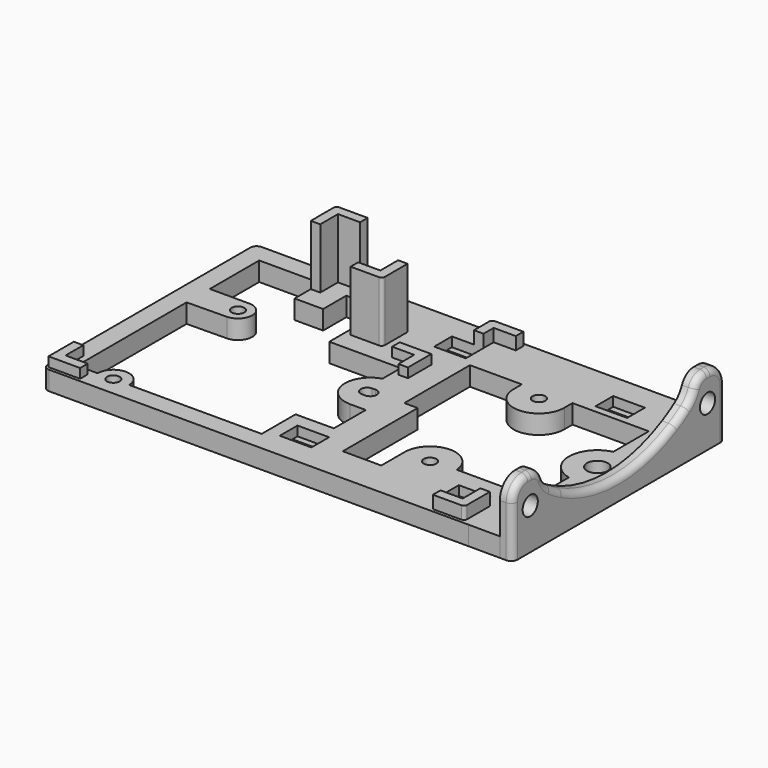
from build123d import *

# Parameters (mm, degrees)
F0_R      = 2
F0_R_2    = 3.3
F1_DEPTH  = 6
F2_DEPTH  = 10
F3_R      = 3
F4_DEPTH  = 4
F5_R      = 5
F6_R      = 5
F7_R      = 6
F8_R      = 6
F9_DEPTH  = 25
F0_W      = 10
F0_H      = 2
F10_DEPTH = 3
F11_R     = 2
F12_R     = 1
F14_DEPTH = 9


# Not quite as in the source:
# - two fillets or chamfers of one size are made in one step
# - a feature names something its author has since deleted; it is built from what else it names


with BuildPart() as f1:
    # F0 (on Top) → F1 (new body)
    with BuildSketch(Plane.XY):
        with BuildLine():
            Line((-86.7564441767, -23.0754980175), (-72.2564441767, -23.0754980175))
            Line((-72.2564441767, -23.0754980175), (47.7435558233, -23.0754980175))
            Line((47.7435558233, -23.0754980175), (57.7435558233, -23.1136400253))
            Line((57.7435558233, -23.1136400253), (57.7435558233, 60.9245019825))
            Line((57.7435558233, 60.9245019825), (47.7435558233, 60.9245019825))
            Line((47.7435558233, 60.9245019825), (-51.2561814487, 60.9245019825))
            Line((-51.2561814487, 60.9245019825), (-51.2561814487, 57.9245019825))
            Line((-51.2561814487, 57.9245019825), (-58.2561814487, 57.9245019825))
            Line((-58.2561814487, 57.9245019825), (-58.2561814487, 50.9245019825))
            Line((-58.2561814487, 50.9245019825), (-61.2395893335, 50.9245019825))
            Line((-61.2395893335, 50.9245019825), (-61.2395893335, 44.5048203142))
            Line((-61.2395893335, 44.5048203142), (-52.2176701128, 44.5048203142))
            Line((-52.2176701128, 44.5048203142), (-52.2176701128, 53.653809187))
            Line((-52.2176701128, 53.653809187), (-40.1129797101, 53.653809187))
            Line((-40.1129797101, 53.653809187), (-40.1129797101, 31.8128021718))
            Line((-40.1129797101, 31.8128021718), (-17.5129008609, 31.8128021718))
            Line((-17.5129008609, 31.8128021718), (-17.5129008609, 24.5912035212))
            ThreePointArc((-17.5129008609, 24.5912035212), (-23.1431978211, 15.7845076931), (-15.238202653, 8.9457076039))
            Line((-15.238202653, 8.9457076039), (-10.2788253924, 8.9457076039))
            Line((-10.2788253924, 8.9457076039), (-10.3093263865, -3.6202194019))
            Line((-10.3093263865, -3.6202194019), (-17.5720681512, -3.6837886869))
            Line((-17.5720681512, -3.6837886869), (-22.366784513, -3.6837886869))
            Line((-22.366784513, -3.6837886869), (-22.366784513, -17.0754980175))
            Line((-22.366784513, -17.0754980175), (-64.2564441767, -17.0754980175))
            ThreePointArc((-64.2564441767, -17.0754980175), (-69.2564441767, -12.0754980175), (-74.2564441767, -17.0754980175))
            Line((-74.2564441767, -17.0754980175), (-80.7564441767, -17.0754980175))
            Line((-80.7564441767, -17.0754980175), (-80.7564441767, 25.9245019825))
            Line((-80.7564441767, 25.9245019825), (-80.7564441767, 26.241465704))
            Line((-80.7564441767, 26.241465704), (-68.1906985893, 26.4228306818))
            ThreePointArc((-68.1906985893, 26.4228306818), (-63.7557587674, 30.9548343886), (-68.2556416043, 35.4223620357))
            Line((-68.2556416043, 35.4223620357), (-80.7564441767, 35.4223620357))
            Line((-80.7564441767, 35.4223620357), (-80.7564441767, 39.9245019825))
            Line((-80.7564441767, 39.9245019825), (-80.7564441767, 54.9245019825))
            Line((-80.7564441767, 54.9245019825), (-61.2561814487, 54.9245019825))
            Line((-61.2561814487, 54.9245019825), (-61.2561814487, 60.9245019825))
            Line((-61.2561814487, 60.9245019825), (-72.2564441767, 60.9245019825))
            Line((-72.2564441767, 60.9245019825), (-86.7564441767, 60.9245019825))
            Line((-86.7564441767, 60.9245019825), (-86.7564441767, -23.0754980175))
        make_face()
        Polygon((-85.7564441767, -22.0754980175), (-85.7564441767, -12.0754980175), (-82.7564441767, -12.0754980175), (-82.7564441767, -19.0754980175), (-75.7564441767, -19.0754980175), (-75.7564441767, -22.0754980175), align=None, mode=Mode.SUBTRACT)
        with Locations((-69.2564441767, -17.0754980175)):
            Circle(F0_R, mode=Mode.SUBTRACT)
        with BuildLine():
            ThreePointArc((-15.238202653, 18.9431274506), (-13.228889919, 16.9338147165), (-15.238202653, 14.9245019825))
            Line((-15.238202653, 14.9245019825), (-16.2564441767, 14.9245019825))
            ThreePointArc((-16.2564441767, 14.9245019825), (-18.2566361489, 16.9429354784), (-16.238202653, 18.9431274506))
            Line((-16.238202653, 18.9431274506), (-15.238202653, 18.9431274506))
        make_face(mode=Mode.SUBTRACT)
        Polygon((-18.2564441767, -8.0754980175), (-8.2564441767, -8.0754980175), (-8.2564441767, -10.0754980175), (-8.2564441767, -13.0754980175), (-8.2564441767, -15.0754980175), (-18.2564441767, -15.0754980175), (-18.2564441767, -13.0754980175), (-18.2564441767, -10.0754980175), align=None, mode=Mode.SUBTRACT)
        with Locations((19.2435558233, -2.5754980175)):
            Circle(F0_R, mode=Mode.SUBTRACT)
        Polygon((35.7435558233, -22.0754980175), (35.7435558233, -19.0754980175), (42.7435558233, -19.0754980175), (42.7435558233, -15.0754980175), (32.7435558233, -15.0754980175), (32.7435558233, -13.0754980175), (32.7435558233, -10.0754980175), (32.7435558233, -8.0754980175), (42.7435558233, -8.0754980175), (42.7435558233, -10.0754980175), (42.7435558233, -12.0754980175), (45.7435558233, -12.0754980175), (45.7435558233, -22.0754980175), align=None, mode=Mode.SUBTRACT)
        with BuildLine():
            Line((-5.1740920527, 17.7788819765), (-5.1740920527, 43.6987291669))
            Line((-5.1740920527, 43.6987291669), (11.2468365315, 43.6987291669))
            Line((11.2468365315, 43.6987291669), (11.2468365315, 40.6535883589))
            ThreePointArc((11.2468365315, 40.6535883589), (19.1805386507, 32.4247501841), (27.2428917132, 40.5275811782))
            Line((27.2428917132, 40.5275811782), (27.2428917132, 43.6987291669))
            Line((27.2428917132, 43.6987291669), (51.374650299, 43.6987291669))
            Line((51.374650299, 43.6987291669), (51.374650299, 29.6435850184))
            ThreePointArc((51.374650299, 29.6435850184), (44.374650299, 20.868620631), (51.374650299, 12.0936562436))
            Line((51.374650299, 12.0936562436), (51.374650299, -1.9614879048))
            Line((51.374650299, -1.9614879048), (27.2199579936, -1.9614879048))
            ThreePointArc((27.2199579936, -1.9614879048), (18.9363241209, 5.4186003482), (11.2435558233, -2.5754980175))
            Line((11.2435558233, -2.5754980175), (11.2435558233, -11.83494631))
            Line((11.2435558233, -11.83494631), (-0.9362465127, -11.83494631))
            Line((-0.9362465127, -11.83494631), (-0.9362465127, -5.9105487922))
            Line((-0.9362465127, -5.9105487922), (-0.9362465127, 17.7788819765))
            Line((-0.9362465127, 17.7788819765), (-5.1740920527, 17.7788819765))
        make_face(mode=Mode.SUBTRACT)
        with Locations((-68.2556416043, 30.9223620357)):
            Circle(F0_R, mode=Mode.SUBTRACT)
        Polygon((-15.7564441767, 34.9245019825), (-22.7564441767, 34.9245019825), (-22.7564441767, 37.9245019825), (-12.7564441767, 37.9245019825), (-12.7564441767, 28.7011023611), (-15.7564441767, 28.7011023611), align=None, mode=Mode.SUBTRACT)
        Polygon((-38.2561814487, 37.9245019825), (-38.2561814487, 40.9245019825), (-31.2561814487, 40.9245019825), (-31.2561814487, 47.9245019825), (-28.2561814487, 47.9245019825), (-28.2561814487, 37.9245019825), align=None, mode=Mode.SUBTRACT)
        with Locations((53.374650299, 20.868620631)):
            Circle(F0_R_2, mode=Mode.SUBTRACT)
        with Locations((19.2435558233, 40.4245019825)):
            Circle(F0_R, mode=Mode.SUBTRACT)
        Polygon((-1.2564441767, 59.9245019825), (-1.2564441767, 56.9245019825), (-8.2564441767, 56.9245019825), (-8.2564441767, 52.9245019825), (-8.2564441767, 50.9245019825), (-8.2564441767, 49.9245019825), (-8.2564441767, 47.9245019825), (-8.2564441767, 45.9245019825), (-18.2564441767, 45.9245019825), (-18.2564441767, 47.9245019825), (-18.2564441767, 50.9245019825), (-18.2564441767, 52.9245019825), (-11.2564441767, 52.9245019825), (-11.2564441767, 59.9245019825), align=None, mode=Mode.SUBTRACT)
        Polygon((32.7435558233, 52.9245019825), (42.7435558233, 52.9245019825), (42.7435558233, 50.9245019825), (42.7435558233, 47.9245019825), (42.7435558233, 45.9245019825), (32.7435558233, 45.9245019825), (32.7435558233, 47.9245019825), (32.7435558233, 50.9245019825), align=None, mode=Mode.SUBTRACT)
    extrude(amount=F1_DEPTH)

    # F0 (on Top) → F2 (join)
    with BuildSketch(Plane.XY):
        Polygon((-8.2564441767, 56.9245019825), (-1.2564441767, 56.9245019825), (-1.2564441767, 59.9245019825), (-11.2564441767, 59.9245019825), (-11.2564441767, 52.9245019825), (-8.2564441767, 52.9245019825), align=None)
        Polygon((42.7435558233, -19.0754980175), (35.7435558233, -19.0754980175), (35.7435558233, -22.0754980175), (45.7435558233, -22.0754980175), (45.7435558233, -12.0754980175), (42.7435558233, -12.0754980175), (42.7435558233, -13.0754980175), (42.7435558233, -15.0754980175), align=None)
    extrude(amount=F2_DEPTH)

    # F3 (on face) → F4 (join)
    with BuildSketch(Plane.YZ.offset(57.7435558233)):
        with BuildLine():
            Line((-23.1136400253, 22), (-23.1136400253, 6))
            Line((-23.1136400253, 6), (-3.1136400253, 6))
            Line((-3.1136400253, 6), (-3.1136400253, 12.0944824391))
            ThreePointArc((-3.1136400253, 12.0944824391), (-5.5611228252, 13.4716458983), (-7.9227862343, 14.9912830889))
            ThreePointArc((-7.9227862343, 14.9912830889), (-10.634535676, 18.0394282469), (-11.6136400253, 22))
            Line((-11.6136400253, 22), (-23.1136400253, 22))
        make_face()
        with Locations((-16.1136400253, 13)):
            Circle(F3_R, mode=Mode.SUBTRACT)
        Polygon((-23.1136400253, 6), (-23.1136400253, 0), (60.9245019825, 0), (60.9245019825, 6), (40.9245019825, 6), (-3.1136400253, 6), align=None)
        with BuildLine():
            Line((-3.1136400253, 12.0944824391), (-3.1136400253, 6))
            Line((-3.1136400253, 6), (40.9245019825, 6))
            Line((40.9245019825, 6), (40.9245019825, 12.0944824391))
            ThreePointArc((40.9245019825, 12.0944824391), (18.9054309786, 6.6720378641), (-3.1136400253, 12.0944824391))
        make_face()
        with BuildLine():
            Line((40.9245019825, 6), (60.9245019825, 6))
            Line((60.9245019825, 6), (60.9245019825, 22))
            Line((60.9245019825, 22), (49.4245019825, 22))
            ThreePointArc((49.4245019825, 22), (48.4453976332, 18.0394282469), (45.7336481916, 14.9912830889))
            ThreePointArc((45.7336481916, 14.9912830889), (43.3719847825, 13.4716458983), (40.9245019825, 12.0944824391))
            Line((40.9245019825, 12.0944824391), (40.9245019825, 6))
        make_face()
        with Locations((53.9245019825, 13)):
            Circle(F3_R, mode=Mode.SUBTRACT)
    extrude(amount=F4_DEPTH)

    # F5
    f5_edges = [f1.edges().sort_by_distance(p)[0] for p in [
        (59.743556, -11.61364, 22),
    ]]
    fillet(f5_edges, radius=F5_R)

    # F6
    f6_edges = [f1.edges().sort_by_distance(p)[0] for p in [
        (59.743556, 49.424502, 22),
    ]]
    fillet(f6_edges, radius=F6_R)

    # F7
    f7_edges = [f1.edges().sort_by_distance(p)[0] for p in [
        (59.743556, 60.924502, 22),
    ]]
    fillet(f7_edges, radius=F7_R)

    # F8
    f8_edges = [f1.edges().sort_by_distance(p)[0] for p in [
        (59.743556, -23.11364, 22),
    ]]
    fillet(f8_edges, radius=F8_R)

    # F0 (on Top) → F9 (join)
    with BuildSketch(Plane.XY):
        Polygon((-51.2561814487, 60.9245019825), (-61.2561814487, 60.9245019825), (-61.2561814487, 54.9245019825), (-61.2395893335, 54.9245019825), (-61.2395893335, 50.9245019825), (-58.2561814487, 50.9245019825), (-58.2561814487, 57.9245019825), (-51.2561814487, 57.9245019825), align=None)
        Polygon((-31.2561814487, 40.9245019825), (-38.2561814487, 40.9245019825), (-38.2561814487, 37.9245019825), (-28.2561814487, 37.9245019825), (-28.2561814487, 47.9245019825), (-31.2561814487, 47.9245019825), align=None)
    extrude(amount=F9_DEPTH)

    # F0 (on Top) → F10 (join)
    with BuildSketch(Plane.XY):
        Polygon((-8.2564441767, 50.9245019825), (-8.2564441767, 52.9245019825), (-11.2564441767, 52.9245019825), (-18.2564441767, 52.9245019825), (-18.2564441767, 50.9245019825), align=None)
        with Locations((-13.2564441767, 46.9245019825)):
            Rectangle(F0_W, F0_H)
        with Locations((37.7435558233, 51.9245019825)):
            Rectangle(F0_W, F0_H)
        with Locations((37.7435558233, 46.9245019825)):
            Rectangle(F0_W, F0_H)
        with Locations((37.7435558233, -9.0754980175)):
            Rectangle(F0_W, F0_H)
        with Locations((37.7435558233, -14.0754980175)):
            Rectangle(F0_W, F0_H)
        with Locations((-13.2564441767, -14.0754980175)):
            Rectangle(F0_W, F0_H)
        with Locations((-13.2564441767, -9.0754980175)):
            Rectangle(F0_W, F0_H)
    extrude(amount=F10_DEPTH)

    # F11
    f11_edges = [f1.edges().sort_by_distance(p)[0] for p in [
        (-86.756444, -23.075498, 3),
        (61.743556, -23.11364, 8),
        (61.743556, -21.356281, 20.242641),
        (61.743556, -16.383608, 22),
        (61.743556, 60.924502, 8),
        (-86.756444, 60.924502, 3),
        (61.743556, -12.848158, 21.138796),
        (61.743556, 59.167143, 20.242641),
        (61.743556, -9.752774, 16.69228),
        (61.743556, 54.19447, 22),
        (61.743556, 18.905431, 6.672038),
        (61.743556, 50.65902, 21.138796),
        (61.743556, 47.563636, 16.69228),
    ]]
    fillet(f11_edges, radius=F11_R)

    # F12
    f12_edges = [f1.edges().sort_by_distance(p)[0] for p in [
        (-11.256444, 59.924502, 8),
        (-61.256181, 60.924502, 15.5),
        (45.743556, -22.075498, 8),
        (-28.256181, 37.924502, 15.5),
    ]]
    fillet(f12_edges, radius=F12_R)

    # F0 (on Top) → F14 (join)
    with BuildSketch(Plane.XY):
        Polygon((-82.7564441767, -12.0754980175), (-85.7564441767, -12.0754980175), (-85.7564441767, -22.0754980175), (-75.7564441767, -22.0754980175), (-75.7564441767, -19.0754980175), (-82.7564441767, -19.0754980175), align=None)
        Polygon((-22.7564441767, 37.9245019825), (-22.7564441767, 34.9245019825), (-15.7564441767, 34.9245019825), (-15.7564441767, 28.7011023611), (-12.7564441767, 28.7011023611), (-12.7564441767, 37.9245019825), align=None)
    extrude(amount=F14_DEPTH)


solid = f1.part
